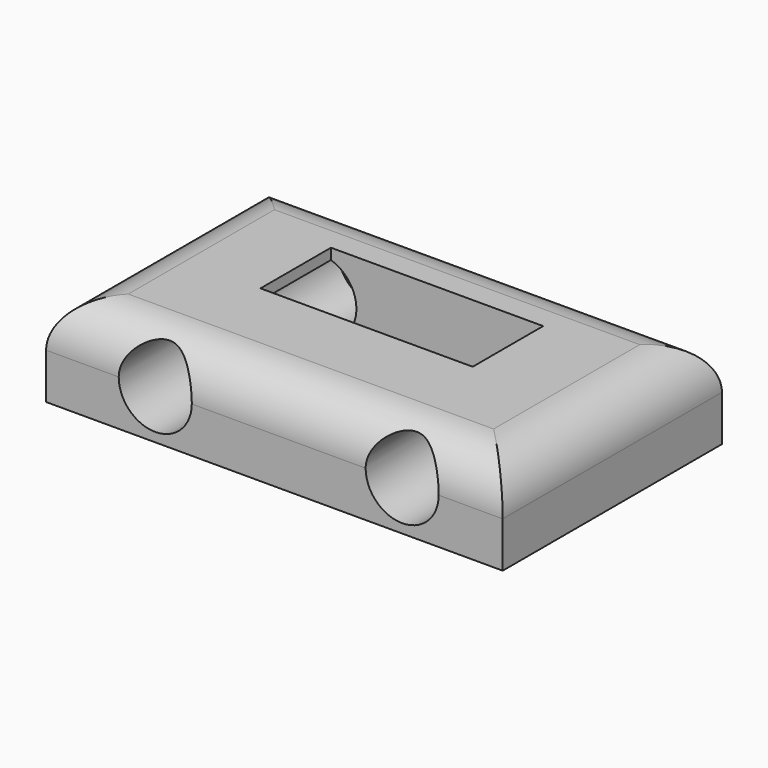
from build123d import *

# Parameters (mm, degrees)
F0_W        = 50
F0_H        = 10
F1_DEPTH    = 30
F3_D        = 8
F4_T1_DEPTH = 55
F4_T3_DEPTH = 75
F5_W        = 23.234388791
F5_H        = 9.6455635503
F6_DEPTH    = 25


# Not quite as in the source:
# - a fillet or chamfer that OpenCascade refuses, or shapes differently, is made with other operations: its cross-section is extruded or revolved along the edge and cut away or added


with BuildPart() as f1:
    # F0 (on Front) → F1 (new body)
    with BuildSketch(Plane.XZ):
        Rectangle(F0_W, F0_H)
    extrude(amount=F1_DEPTH)

    # F3 (through all)
    with Locations(Plane(origin=(0, 0, 0), x_dir=(1, 0, 0), z_dir=(0, 1, 0))):
        with Locations((-13.0464080721, 0), (13.9895221218, 0)):
            Hole(F3_D / 2)

    # F4: fillet of radius 5 on 4 edges, made by hand

    # F4_s2 → F4_t1 (cut)
    with BuildSketch(Plane.XZ.offset(-12.5)):
        with BuildLine():
            ThreePointArc((20, 5), (23.5355339059, 3.5355339059), (25, 0))
            Line((25, 0), (25, 5))
            Line((25, 5), (20, 5))
        make_face()
        with BuildLine():
            ThreePointArc((-20, 5), (-23.5355339059, 3.5355339059), (-25, 0))
            Line((-25, 0), (-25, 5))
            Line((-25, 5), (-20, 5))
        make_face()
    extrude(amount=F4_T1_DEPTH, mode=Mode.SUBTRACT)

    # F4_s4 → F4_t3 (cut)
    with BuildSketch(Plane.YZ.offset(-37.5)):
        with BuildLine():
            ThreePointArc((-5, 5), (-1.4644660941, 3.5355339059), (0, 0))
            Line((0, 0), (0, 5))
            Line((0, 5), (-5, 5))
        make_face()
        with BuildLine():
            ThreePointArc((-25, 5), (-28.5355339059, 3.5355339059), (-30, 0))
            Line((-30, 0), (-30, 5))
            Line((-30, 5), (-25, 5))
        make_face()
    extrude(amount=F4_T3_DEPTH, mode=Mode.SUBTRACT)

    # F5 (on face) → F6 (cut)
    with BuildSketch(Plane.XY.offset(5)):
        with Locations((-0.2135247923, -12.2946440242)):
            Rectangle(F5_W, F5_H)
    extrude(amount=-F6_DEPTH, mode=Mode.SUBTRACT)


solid = f1.part
